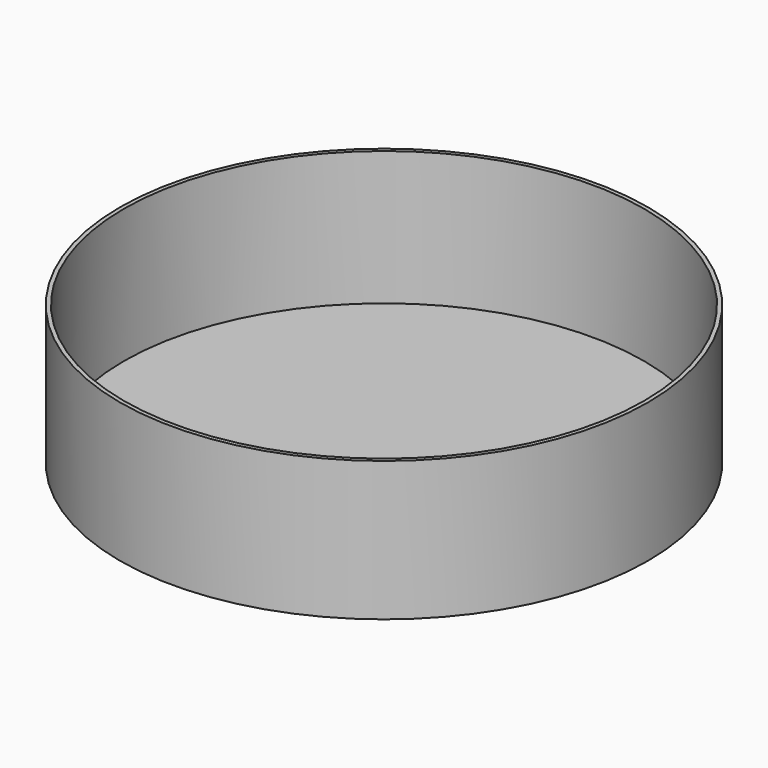
from build123d import *

# Parameters (mm, degrees)
F0_R         = 49.25
F0_R_2       = 48.5
F1_DEPTH     = 2
F2_DEPTH     = 25
F3_R         = 49.25
F3_W         = 2.8827052956
F3_H         = 13.592446332
F3_TEXT_SIZE = 19.0395396203
F4_DEPTH     = 1


# Not quite as in the source:
# - Text() gives the source's letters only with a copy of the font that has no kerning and outlines rounded to 1/6400 em; it was checked with that copy


with BuildPart() as f1:
    # F0 (on Top) → F1 (new body)
    with BuildSketch(Plane.XY):
        Circle(F0_R)
        Circle(F0_R_2, mode=Mode.SUBTRACT)
        Circle(F0_R_2)
    extrude(amount=-F1_DEPTH)

    # F0 (on Top) → F2 (join)
    with BuildSketch(Plane.XY):
        Circle(F0_R)
        Circle(F0_R_2, mode=Mode.SUBTRACT)
    extrude(amount=F2_DEPTH)

    # F3 (on face) → F4 (cut)
    with BuildSketch(Plane(origin=(0, 0, -2), x_dir=(1, 0, 0), z_dir=(0, 0, -1))):
        Circle(F3_R)
        with BuildLine():
            Line((-16.2193066499, 25.6532618005), (-16.2193066499, 12.0608154684))
            Line((-16.2193066499, 12.0608154684), (-19.8814430987, 12.0608154684))
            Line((-19.8814430987, 12.0608154684), (-25.7956000933, 22.3421668634))
            Line((-25.7956000933, 22.3421668634), (-25.8788980791, 22.3421668634))
            add(Edge.make_bspline(
                [(-25.8788980791, 22.3421668634), (-25.7004023952, 19.6201076833), (-25.7004023952, 18.4569108096)],
                knots=[0, 0, 0, 1, 1, 1], degree=2))
            Line((-25.7004023952, 18.4569108096), (-25.7004023952, 12.0608154684))
            Line((-25.7004023952, 12.0608154684), (-28.2766901, 12.0608154684))
            Line((-28.2766901, 12.0608154684), (-28.2766901, 25.6532618005))
            Line((-28.2766901, 25.6532618005), (-24.6413280038, 25.6532618005))
            Line((-24.6413280038, 25.6532618005), (-18.7390707215, 15.4730579598))
            Line((-18.7390707215, 15.4730579598), (-18.673622304, 15.4730579598))
            add(Edge.make_bspline(
                [(-18.673622304, 15.4730579598), (-18.8134439231, 18.1237188663), (-18.8134439231, 19.2184923944)],
                knots=[0, 0, 0, 1, 1, 1], degree=2))
            Line((-18.8134439231, 19.2184923944), (-18.8134439231, 25.6532618005))
            Line((-18.8134439231, 25.6532618005), (-16.2193066499, 25.6532618005))
        make_face(mode=Mode.SUBTRACT)
        with Locations((-11.3567867265, 18.8570386345)):
            Rectangle(F3_W, F3_H, mode=Mode.SUBTRACT)
        Polygon((-0.3391406353, 19.6379572517), (4.4385938381, 12.0608154684), (1.1661729659, 12.0608154684), (-2.3948159287, 17.7875519948), (-3.6115615076, 16.9129231435), (-3.6115615076, 12.0608154684), (-6.4942668032, 12.0608154684), (-6.4942668032, 25.6532618005), (-3.6115615076, 25.6532618005), (-3.6115615076, 19.4326872152), (-2.4781139145, 21.0331985145), (1.2048470307, 25.6532618005), (4.4028947013, 25.6532618005), align=None, mode=Mode.SUBTRACT)
        Polygon((7.5444187387, 12.0608154684), (4.4385938381, 12.0608154684), (9.2371528081, 25.7097854337), (12.7594676378, 25.7097854337), (17.5758761761, 12.0608154684), (14.4700512756, 12.0608154684), (13.4853500858, 15.2975372039), (8.5291199284, 15.2975372039), align=None, mode=Mode.SUBTRACT)
        with BuildLine():
            add(Edge.make_bspline(
                [(29.9634766416, 24.0631627494), (31.6234865022, 22.2588688775), (31.6234865022, 18.8763756669)],
                knots=[0, 0, 0, 1, 1, 1], degree=2))
            add(Edge.make_bspline(
                [(31.6234865022, 18.8763756669), (31.6234865022, 15.4998323123), (29.9500894653, 13.6866136563)],
                knots=[0, 0, 0, 1, 1, 1], degree=2))
            add(Edge.make_bspline(
                [(29.9500894653, 13.6866136563), (28.2766924283, 11.8733950003), (25.1530179594, 11.8733950003)],
                knots=[0, 0, 0, 1, 1, 1], degree=2))
            add(Edge.make_bspline(
                [(25.1530179594, 11.8733950003), (22.0293434904, 11.8733950003), (20.3559464535, 13.6866136563)],
                knots=[0, 0, 0, 1, 1, 1], degree=2))
            add(Edge.make_bspline(
                [(20.3559464535, 13.6866136563), (18.6825494166, 15.4998323123), (18.6825494166, 18.8942252353)],
                knots=[0, 0, 0, 1, 1, 1], degree=2))
            add(Edge.make_bspline(
                [(18.6825494166, 18.8942252353), (18.6825494166, 22.2886181582), (20.3604088456, 24.0780373897)],
                knots=[0, 0, 0, 1, 1, 1], degree=2))
            add(Edge.make_bspline(
                [(20.3604088456, 24.0780373897), (22.0382682746, 25.8674566212), (25.1708675278, 25.8674566212)],
                knots=[0, 0, 0, 1, 1, 1], degree=2))
            add(Edge.make_bspline(
                [(25.1708675278, 25.8674566212), (28.3034667809, 25.8674566212), (29.9634766416, 24.0631627494)],
                knots=[0, 0, 0, 1, 1, 1], degree=2))
        make_face(mode=Mode.SUBTRACT)
        with BuildLine():
            add(Edge.make_bspline(
                [(10.1668178286, 27.5616781546), (9.823213637, 27.71488695), (9.4870467656, 27.71488695)],
                knots=[0, 0, 0, 1, 1, 1], degree=2))
            add(Edge.make_bspline(
                [(9.4870467656, 27.71488695), (9.1984787432, 27.71488695), (8.9337101454, 27.4694553846)],
                knots=[0, 0, 0, 1, 1, 1], degree=2))
            add(Edge.make_bspline(
                [(8.9337101454, 27.4694553846), (8.6689415475, 27.2240238191), (8.5499444249, 26.721260976)],
                knots=[0, 0, 0, 1, 1, 1], degree=2))
            Line((8.5499444249, 26.721260976), (7.1636279463, 26.721260976))
            add(Edge.make_bspline(
                [(7.1636279463, 26.721260976), (7.2647755005, 28.0689033898), (7.9296719232, 28.8319724386)],
                knots=[0, 0, 0, 1, 1, 1], degree=2))
            add(Edge.make_bspline(
                [(7.9296719232, 28.8319724386), (8.5945683459, 29.5950414875), (9.6923168021, 29.5950414875)],
                knots=[0, 0, 0, 1, 1, 1], degree=2))
            add(Edge.make_bspline(
                [(9.6923168021, 29.5950414875), (10.0731075945, 29.5950414875), (10.4405112106, 29.4403452281)],
                knots=[0, 0, 0, 1, 1, 1], degree=2))
            add(Edge.make_bspline(
                [(10.4405112106, 29.4403452281), (10.8079148267, 29.2856489687), (11.1663936586, 29.1056658207)],
                knots=[0, 0, 0, 1, 1, 1], degree=2))
            add(Edge.make_bspline(
                [(11.1663936586, 29.1056658207), (11.5248724906, 28.9256826727), (11.8684766821, 28.7769362694)],
                knots=[0, 0, 0, 1, 1, 1], degree=2))
            add(Edge.make_bspline(
                [(11.8684766821, 28.7769362694), (12.2120808737, 28.6281898661), (12.5452728171, 28.6281898661)],
                knots=[0, 0, 0, 1, 1, 1], degree=2))
            add(Edge.make_bspline(
                [(12.5452728171, 28.6281898661), (12.8338408394, 28.6281898661), (13.0986094373, 28.8691590395)],
                knots=[0, 0, 0, 1, 1, 1], degree=2))
            add(Edge.make_bspline(
                [(13.0986094373, 28.8691590395), (13.3633780351, 29.1101282128), (13.4853500858, 29.6128910559)],
                knots=[0, 0, 0, 1, 1, 1], degree=2))
            Line((13.4853500858, 29.6128910559), (14.8716665644, 29.6128910559))
            add(Edge.make_bspline(
                [(14.8716665644, 29.6128910559), (14.7675440821, 28.2652486421), (14.0937228753, 27.5021795933)],
                knots=[0, 0, 0, 1, 1, 1], degree=2))
            add(Edge.make_bspline(
                [(14.0937228753, 27.5021795933), (13.4199016684, 26.7391105444), (12.3429777086, 26.7391105444)],
                knots=[0, 0, 0, 1, 1, 1], degree=2))
            add(Edge.make_bspline(
                [(12.3429777086, 26.7391105444), (11.9592119881, 26.7391105444), (11.5932958361, 26.8923193398)],
                knots=[0, 0, 0, 1, 1, 1], degree=2))
            add(Edge.make_bspline(
                [(11.5932958361, 26.8923193398), (11.227379684, 27.0455281352), (10.8689008521, 27.2269987472)],
                knots=[0, 0, 0, 1, 1, 1], degree=2))
            add(Edge.make_bspline(
                [(10.8689008521, 27.2269987472), (10.5104220202, 27.4084693592), (10.1668178286, 27.5616781546)],
                knots=[0, 0, 0, 1, 1, 1], degree=2))
        make_face(mode=Mode.SUBTRACT)
        with Locations((-29.9872737378, 12.0608154684)):
            Text('NIKÃO', F3_TEXT_SIZE, font='Open Sans', font_style=FontStyle.BOLD, text_align=(TextAlign.LEFT, TextAlign.BOTTOM))
    extrude(amount=-F4_DEPTH, mode=Mode.SUBTRACT)


solid = f1.part
